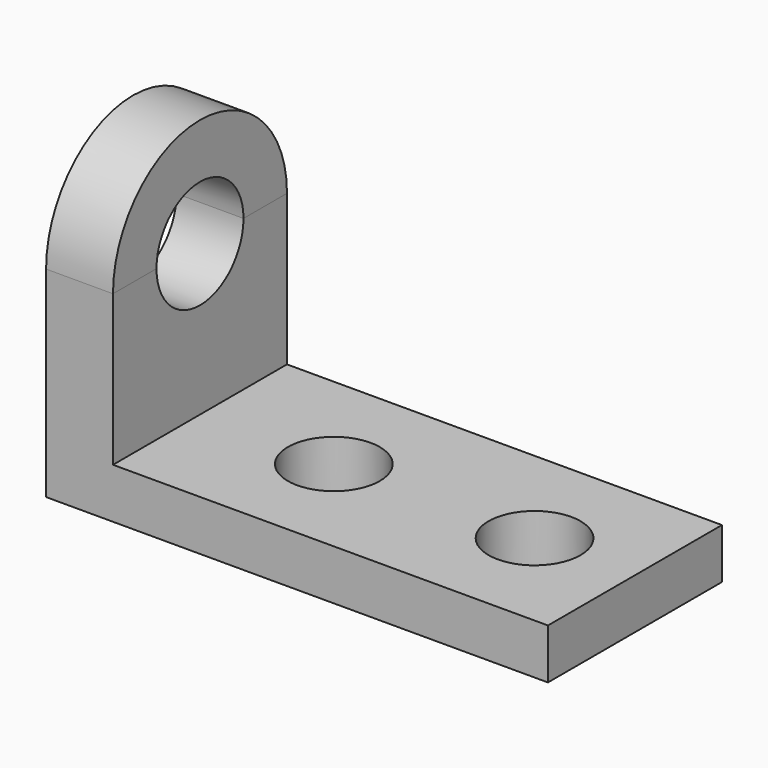
from build123d import *

# Parameters (mm, degrees)
F0_W      = 190.5
F0_H      = 82.55
F1_DEPTH  = 19.05
F2_W      = 25.4
F2_H      = 82.55
F3_DEPTH  = 57.15
F5_DEPTH  = 25.4
F7_DEPTH  = 25.4
F9_DEPTH  = 25.4
F10_R     = 17.4625
F11_DEPTH = 25.4
F12_R     = 17.4625
F13_DEPTH = 25.4


with BuildPart() as f1:
    # F0 (on Top) → F1 (new body)
    with BuildSketch(Plane.XY):
        with Locations((51.8731928766, 3.7849264085)):
            Rectangle(F0_W, F0_H)
    extrude(amount=F1_DEPTH)

    # F2 (on face) → F3 (join)
    with BuildSketch(Plane.XY.offset(19.05)):
        with Locations((-30.6768071234, 3.7849264085)):
            Rectangle(F2_W, F2_H)
    extrude(amount=F3_DEPTH)


with BuildPart() as f5:
    # F4 (on face) → F5 (new body)
    with BuildSketch(Plane.YZ.offset(-17.9768071234)):
        with BuildLine():
            Line((-37.4900735915, 76.2), (45.0599264085, 76.2))
            ThreePointArc((45.0599264085, 76.2), (3.7849264085, 117.475), (-37.4900735915, 76.2))
        make_face()
    extrude(amount=-F5_DEPTH)


with BuildPart() as f7_tool:
    # F6 (on face) → F7 (new body)
    with BuildSketch(Plane.YZ.offset(-17.9768071234)):
        with BuildLine():
            Line((-16.8525735915, 76.2), (24.4224264085, 76.2))
            ThreePointArc((24.4224264085, 76.2), (3.7849264085, 96.8375), (-16.8525735915, 76.2))
        make_face()
        with BuildLine():
            ThreePointArc((-16.8525735915, 76.2), (3.7849264085, 55.5625), (24.4224264085, 76.2))
            Line((24.4224264085, 76.2), (-16.8525735915, 76.2))
        make_face()
    extrude(amount=-F7_DEPTH)


with BuildPart() as f1_1:
    add(f1.part)

    # F7: cut by f7_tool
    add(f7_tool.part, mode=Mode.SUBTRACT)

    # F8 (on face) → F9 (cut)
    with BuildSketch(Plane.YZ.offset(-17.9768071234)):
        with BuildLine():
            ThreePointArc((-16.8525735915, 76.2), (3.7849264085, 55.5625), (24.4224264085, 76.2))
            ThreePointArc((24.4224264085, 76.2), (3.7849264085, 96.8375), (-16.8525735915, 76.2))
        make_face()
    extrude(amount=-F9_DEPTH, mode=Mode.SUBTRACT)

    # F10 (on face) → F11 (cut)
    with BuildSketch(Plane.XY.offset(19.05)):
        with Locations((109.0231928766, 3.7849264085)):
            Circle(F10_R)
    extrude(amount=-F11_DEPTH, mode=Mode.SUBTRACT)

    # F12 (on face) → F13 (cut)
    with BuildSketch(Plane.XY.offset(19.05)):
        with Locations((32.8231928766, 3.7849264085)):
            Circle(F12_R)
    extrude(amount=-F13_DEPTH, mode=Mode.SUBTRACT)


with BuildPart() as f5_1:
    add(f5.part)

    # F7: cut by f7_tool
    add(f7_tool.part, mode=Mode.SUBTRACT)


solid = Compound([f1_1.part, f5_1.part])
